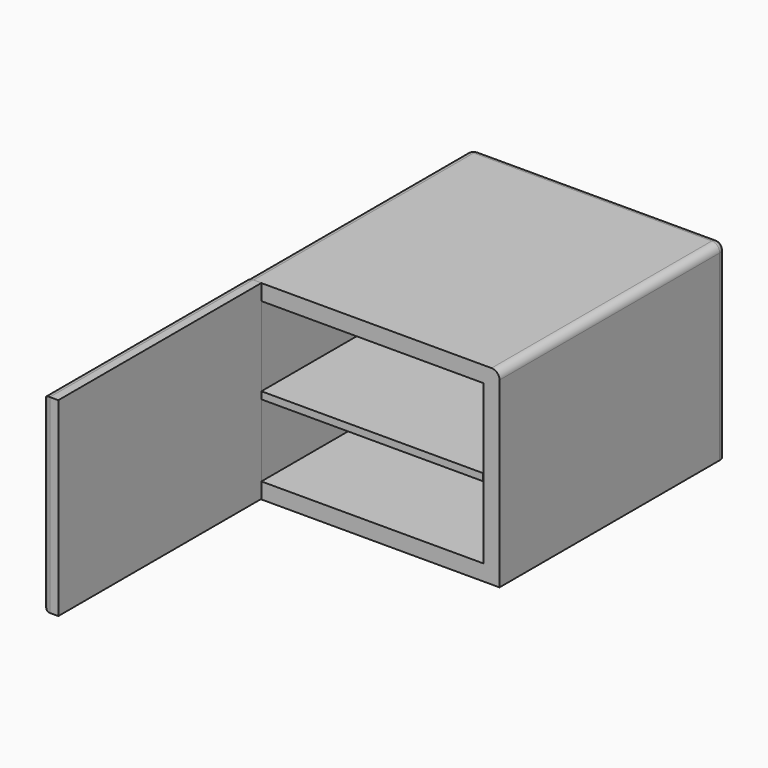
from build123d import *

# Parameters (mm, degrees)
F0_W         = 160
F0_H         = 120
F0_W_2       = 140
F0_H_2       = 100
F1_DEPTH     = 153.4
F2_W         = 160
F2_H         = 120
F3_DEPTH     = 25
F5_W         = 3
F5_H         = 25
F5_W_2       = 2.5065724061
F5_H_2       = 21.7677888939
F7_W         = 10.3015974164
F7_H         = 119.727473706
F8_DEPTH     = 160
F9_R         = 10.5745800983
F10_DEPTH    = 5
F11_W        = 7
F11_H        = 7
F12_DEPTH    = 21.1
F13_R        = 2.005862126
F14_DEPTH    = 20
F15_R        = 2.1
F16_DEPTH    = 20
F17_R        = 2.1
F18_DEPTH    = 20
F19_R        = 2.218699255
F20_DEPTH    = 20
F21_W        = 45
F21_H        = 30
F22_DEPTH    = 5
F23_W        = 35
F23_H        = 7.2088057839
F24_DEPTH    = 5
F25_W        = 8
F25_H        = 3.5
F26_DEPTH    = 5
F27_W        = 140
F27_H        = 4.4944308201
F28_DEPTH    = 176
F29_W        = 29
F29_H        = 3.2
F30_DEPTH    = 5
F31_R        = 5
F32_T1_DEPTH = 185
F32_T3_DEPTH = 144.727473706
F32_T5_DEPTH = 172.5


# Not quite as in the source:
# - a fillet or chamfer that OpenCascade refuses, or shapes differently, is made with other operations: its cross-section is extruded or revolved along the edge and cut away or added


with BuildPart() as f1:
    # F0 (on Front) → F1 (new body)
    with BuildSketch(Plane.XZ):
        Rectangle(F0_W, F0_H)
        Rectangle(F0_W_2, F0_H_2, mode=Mode.SUBTRACT)
    extrude(amount=-F1_DEPTH)

    # F2 (on face) → F3 (join)
    with BuildSketch(Plane(origin=(0, 153.4, 0), x_dir=(-1, 0, 0), z_dir=(0, 1, 0))):
        Rectangle(F2_W, F2_H)
    extrude(amount=F3_DEPTH)

    # F5 (on face) → F6 (revolve)
    with BuildSketch(Plane.XZ):
        with Locations((-75.5, 22.5)):
            Rectangle(F5_W, F5_H)
        with Locations((-75.746713797, -24.116105553)):
            Rectangle(F5_W_2, F5_H_2)
    revolve(axis=Axis((-74, 0, 22.5), (0, 0, -1)))

    # F7 (on face) → F8 (join)
    with BuildSketch(Plane.XZ):
        with Locations((-75.0872157514, 0.2289246768)):
            Rectangle(F7_W, F7_H)
    extrude(amount=F8_DEPTH)

    # F9 (on face) → F10 (join)
    with BuildSketch(Plane(origin=(-80.2380144596, 0, 0), x_dir=(0, -1, 0), z_dir=(-1, 0, 0))):
        with Locations((78.2749652863, 0)):
            Circle(F9_R)
    extrude(amount=F10_DEPTH)

    # F11 (on face) → F12 (join)
    with BuildSketch(Plane(origin=(-85.2380144596, 0, 0), x_dir=(0, -1, 0), z_dir=(-1, 0, 0))):
        with Locations((78.2749652863, 0)):
            Rectangle(F11_W, F11_H)
    extrude(amount=F12_DEPTH)

    # F13 (on face) → F14 (join)
    with BuildSketch(Plane.XY.offset(3.5)):
        with Locations((-102.9334535655, -78.1808274122)):
            Circle(F13_R)
    extrude(amount=F14_DEPTH)

    # F15 (on face) → F16 (join)
    with BuildSketch(Plane(origin=(0, -74.7749652863, 0), x_dir=(-1, 0, 0), z_dir=(0, 1, 0))):
        with Locations((102.8380144596, 0)):
            Circle(F15_R)
    extrude(amount=F16_DEPTH)

    # F17 (on face) → F18 (join)
    with BuildSketch(Plane.XZ.offset(81.7749652863)):
        with Locations((-102.8380144596, 0)):
            Circle(F17_R)
    extrude(amount=F18_DEPTH)

    # F19 (on face) → F20 (join)
    with BuildSketch(Plane(origin=(0, 0, -3.5), x_dir=(1, 0, 0), z_dir=(0, 0, -1))):
        with Locations((-102.7212624934, 78.1562660312)):
            Circle(F19_R)
    extrude(amount=F20_DEPTH)

    # F21 (on face) → F22 (join)
    with BuildSketch(Plane(origin=(-80.2380144596, 0, 0), x_dir=(0, -1, 0), z_dir=(-1, 0, 0))):
        with Locations((32.2962999344, 34.3826470941)):
            Rectangle(F21_W, F21_H)
    extrude(amount=F22_DEPTH)

    # F23 (on face) → F24 (cut)
    with BuildSketch(Plane(origin=(-85.2380144596, 0, 0), x_dir=(0, -1, 0), z_dir=(-1, 0, 0))):
        with Locations((32.0492885076, 42.2782442022)):
            Rectangle(F23_W, F23_H)
    extrude(amount=-F24_DEPTH, mode=Mode.SUBTRACT)

    # F25 (on face) → F26 (join)
    with BuildSketch(Plane(origin=(-85.2380144596, 0, 0), x_dir=(0, -1, 0), z_dir=(-1, 0, 0))):
        with Locations((21.2962999344, 33.4238413102)):
            Rectangle(F25_W, F25_H)
        with Locations((31.7962999344, 33.4238413102)):
            Rectangle(F25_W, F25_H)
        with Locations((42.2962999344, 33.4238413102)):
            Rectangle(F25_W, F25_H)
        with Locations((21.2962999344, 27.9238413102)):
            Rectangle(F25_W, F25_H)
        with Locations((31.7962999344, 27.9238413102)):
            Rectangle(F25_W, F25_H)
        with Locations((42.2962999344, 27.9238413102)):
            Rectangle(F25_W, F25_H)
    extrude(amount=F26_DEPTH)

    # F27 (on face) → F28 (join)
    with BuildSketch(Plane.XZ):
        with Locations((-0.2423568684, -2.24721541)):
            Rectangle(F27_W, F27_H)
    extrude(amount=-F28_DEPTH)

    # F29 (on face) → F30 (join)
    with BuildSketch(Plane(origin=(-85.2380144596, 0, 0), x_dir=(0, -1, 0), z_dir=(-1, 0, 0))):
        with Locations((31.9544213465, 23.1566587463)):
            Rectangle(F29_W, F29_H)
    extrude(amount=F30_DEPTH)

    # F31
    f31_edges = [f1.edges().sort_by_distance(p)[0] for p in [
        (-80, 89.2, 60),
        (0, 178.4, 60),
        (80, 89.2, 60),
        (80, 178.4, 0),
        (-80, 178.4, 0),
    ]]
    fillet(f31_edges, radius=F31_R)

    # F32: fillet of radius 5 on 3 edges, made by hand

    # F32_s2 → F32_t1 (cut)
    with BuildSketch(Plane.XZ.offset(-12.5)):
        with BuildLine():
            ThreePointArc((-75.2380144596, 60.0926615298), (-78.7735483655, 58.6281954357), (-80.2380144596, 55.0926615298))
            Line((-80.2380144596, 55.0926615298), (-80.2380144596, 60.0926615298))
            Line((-80.2380144596, 60.0926615298), (-75.2380144596, 60.0926615298))
        make_face()
    extrude(amount=F32_T1_DEPTH, mode=Mode.SUBTRACT)

    # F32_s4 → F32_t3 (cut)
    with BuildSketch(Plane.XY.offset(-72.1348121762)):
        with BuildLine():
            ThreePointArc((-80.2380144596, -155), (-78.7735483655, -158.5355339059), (-75.2380144596, -160))
            Line((-75.2380144596, -160), (-80.2380144596, -160))
            Line((-80.2380144596, -160), (-80.2380144596, -155))
        make_face()
    extrude(amount=F32_T3_DEPTH, mode=Mode.SUBTRACT)

    # F32_s6 → F32_t5 (cut)
    with BuildSketch(Plane.XZ):
        with BuildLine():
            ThreePointArc((-75.2380144596, -59.6348121762), (-78.7735483655, -58.1703460822), (-80.2380144596, -54.6348121762))
            Line((-80.2380144596, -54.6348121762), (-80.2380144596, -59.6348121762))
            Line((-80.2380144596, -59.6348121762), (-75.2380144596, -59.6348121762))
        make_face()
    extrude(amount=F32_T5_DEPTH, mode=Mode.SUBTRACT)


solid = f1.part
